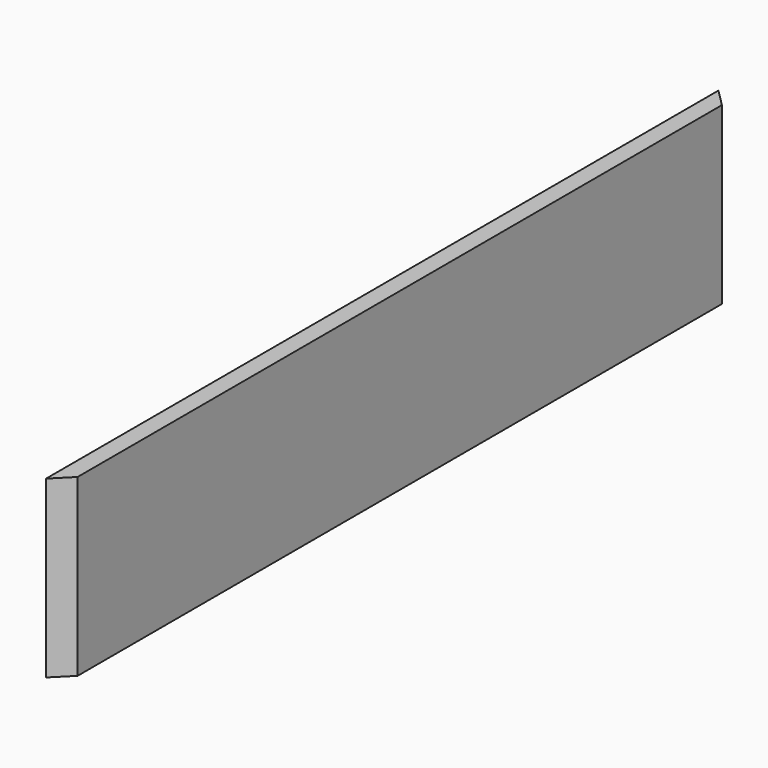
from build123d import *

# Parameters (mm, degrees)
F0_W     = 9.525
F0_H     = 95.25
F1_DEPTH = 457.2
F2_SIZE  = 19.04999


# Not quite as in the source:
# - a fillet or chamfer is up to 0.001 mm smaller than in the source, because OpenCascade refuses the exact size


with BuildPart() as f1:
    # F0 (on Front) → F1 (new body, symmetric)
    with BuildSketch(Plane.XZ):
        Polygon((9.525, 95.25), (-9.525, 95.25), (-9.525, 0), (0, 0), (9.525, 0), align=None)
        with Locations((-4.7625, -47.625)):
            Rectangle(F0_W, F0_H)
        with Locations((4.7625, -47.625)):
            Rectangle(F0_W, F0_H)
    extrude(amount=F1_DEPTH, both=True)

    # F2 (size 19.05 in the source; OpenCascade refuses exactly that, so slightly less here)
    f2_edges = [f1.edges().sort_by_distance(p)[0] for p in [
        (9.525, -457.2, 0),
        (9.525, 457.2, 0),
    ]]
    chamfer(f2_edges, length=F2_SIZE)


solid = f1.part
